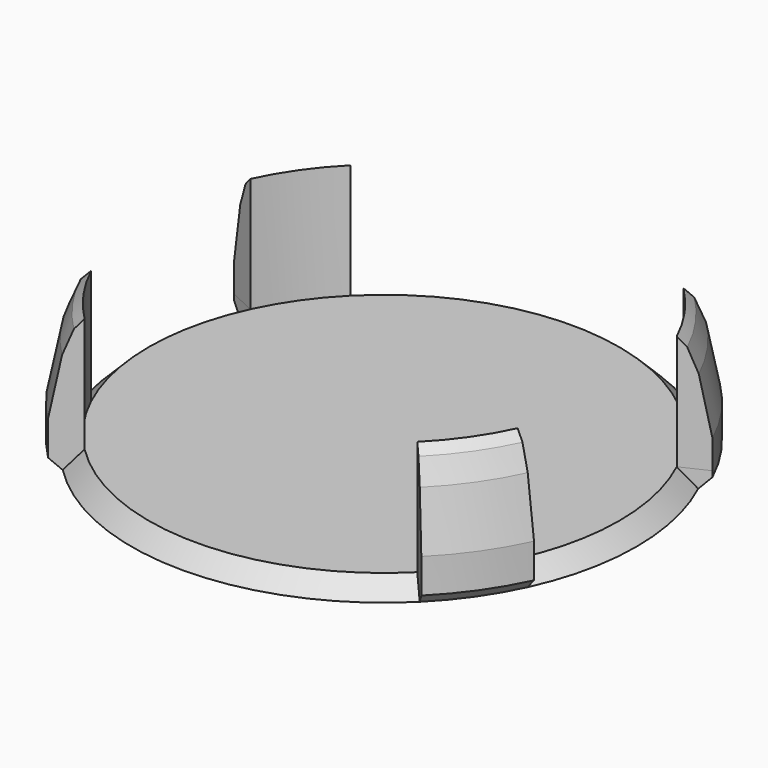
from build123d import *
from build123d import SkipClean  # not in build123d's __all__

# Parameters (mm, degrees)
F1_DEPTH    = 20
F2_SIZE     = 4.99999
F2_2_SIZE   = 4.99999
F2_3_SIZE   = 4.99999
F2_4_SIZE   = 4.99999
F3_DEPTH    = 3
F4_SIZE     = 5
F5_R        = 41
F5_R_2      = 39.2
F6_DEPTH    = 1.5
F7_SIZE     = 5
F8_T2_ANGLE = 50
F8_T4_ANGLE = 90
F8_T6_ANGLE = 50
F8_T8_ANGLE = 90
F9_SIZE     = 2


# Not quite as in the source:
# - a fillet or chamfer that OpenCascade refuses, or shapes differently, is made with other operations: its cross-section is extruded or revolved along the edge and cut away or added
# - a fillet or chamfer is up to 0.001 mm smaller than in the source, because OpenCascade refuses the exact size


with BuildPart() as f1:
    # F0 (on Top) → F1 (new body)
    with BuildSketch(Plane.XY):
        with BuildLine():
            ThreePointArc((-37.1586192685, 17.3273487314), (-33.5852338158, 23.5166338904), (-28.9913780286, 28.9913780286))
            Line((-28.9913780286, 28.9913780286), (-32.5269119346, 32.5269119346))
            ThreePointArc((-32.5269119346, 32.5269119346), (-37.6809940373, 26.3845160721), (-41.6901582037, 19.4404400401))
            Line((-41.6901582037, 19.4404400401), (-37.1586192685, 17.3273487314))
        make_face()
    extrude(amount=F1_DEPTH)

    # F2 (size 5 in the source; OpenCascade refuses exactly that, so slightly less here)
    f2_edges = [f1.edges().sort_by_distance(p)[0] for p in [
        (-37.680994, 26.384516, 20),
    ]]
    chamfer(f2_edges, length=F2_SIZE)



with BuildPart() as f1b:
    # F0 (on Top) → F1, piece 2 (new body)
    with BuildSketch(Plane.XY):
        with BuildLine():
            ThreePointArc((28.9913780286, 28.9913780286), (33.5852338158, 23.5166338904), (37.1586192685, 17.3273487314))
            Line((37.1586192685, 17.3273487314), (41.6901582037, 19.4404400401))
            ThreePointArc((41.6901582037, 19.4404400401), (37.6809940373, 26.3845160721), (32.5269119346, 32.5269119346))
            Line((32.5269119346, 32.5269119346), (28.9913780286, 28.9913780286))
        make_face()
    extrude(amount=F1_DEPTH)

    # F2#2 (size 5 in the source; OpenCascade refuses exactly that, so slightly less here)
    f2_2_edges = [f1b.edges().sort_by_distance(p)[0] for p in [
        (37.680994, 26.384516, 20),
    ]]
    chamfer(f2_2_edges, length=F2_2_SIZE)


with BuildPart() as f1c:
    # F0 (on Top) → F1, piece 3 (new body)
    with BuildSketch(Plane.XY):
        with BuildLine():
            Line((-32.5269119346, -32.5269119346), (-28.9913780286, -28.9913780286))
            ThreePointArc((-28.9913780286, -28.9913780286), (-33.5852338158, -23.5166338904), (-37.1586192685, -17.3273487314))
            Line((-37.1586192685, -17.3273487314), (-41.6901582037, -19.4404400401))
            ThreePointArc((-41.6901582037, -19.4404400401), (-37.6809940373, -26.3845160721), (-32.5269119346, -32.5269119346))
        make_face()
    extrude(amount=F1_DEPTH)

    # F2#3 (size 5 in the source; OpenCascade refuses exactly that, so slightly less here)
    f2_3_edges = [f1c.edges().sort_by_distance(p)[0] for p in [
        (-37.680994, -26.384516, 20),
    ]]
    chamfer(f2_3_edges, length=F2_3_SIZE)


with BuildPart() as f1d:
    # F0 (on Top) → F1, piece 4 (new body)
    with BuildSketch(Plane.XY):
        with BuildLine():
            Line((41.6901582037, -19.4404400401), (37.1586192685, -17.3273487314))
            ThreePointArc((37.1586192685, -17.3273487314), (33.5852338158, -23.5166338904), (28.9913780286, -28.9913780286))
            Line((28.9913780286, -28.9913780286), (32.5269119346, -32.5269119346))
            ThreePointArc((32.5269119346, -32.5269119346), (37.6809940373, -26.3845160721), (41.6901582037, -19.4404400401))
        make_face()
    extrude(amount=F1_DEPTH)

    # F2#4 (size 5 in the source; OpenCascade refuses exactly that, so slightly less here)
    f2_4_edges = [f1d.edges().sort_by_distance(p)[0] for p in [
        (37.680994, -26.384516, 20),
    ]]
    chamfer(f2_4_edges, length=F2_4_SIZE)


with BuildPart() as f1_1:
    add(f1.part, clean=False)

    with SkipClean():  # cleaning this boolean's faces spoils the solid; the shape is the same uncleaned
        add(f1b.part)  # F3 merges F1b

    with SkipClean():  # cleaning this boolean's faces spoils the solid; the shape is the same uncleaned
        add(f1c.part)  # F3 merges F1c

    with SkipClean():  # cleaning this boolean's faces spoils the solid; the shape is the same uncleaned
        add(f1d.part)  # F3 merges F1d
    # F0 (on Top) → F3 (join)
    with BuildSketch(Plane.XY):
        with BuildLine():
            ThreePointArc((-37.1586192685, 17.3273487314), (-33.5852338158, 23.5166338904), (-28.9913780286, 28.9913780286))
            Line((-28.9913780286, 28.9913780286), (-32.5269119346, 32.5269119346))
            ThreePointArc((-32.5269119346, 32.5269119346), (-37.6809940373, 26.3845160721), (-41.6901582037, 19.4404400401))
            Line((-41.6901582037, 19.4404400401), (-37.1586192685, 17.3273487314))
        make_face()
        with BuildLine():
            Line((32.5269119346, -32.5269119346), (28.9913780286, -28.9913780286))
            ThreePointArc((28.9913780286, -28.9913780286), (0, -41), (-28.9913780286, -28.9913780286))
            Line((-28.9913780286, -28.9913780286), (-32.5269119346, -32.5269119346))
            ThreePointArc((-32.5269119346, -32.5269119346), (0, -46), (32.5269119346, -32.5269119346))
        make_face()
        with BuildLine():
            ThreePointArc((28.9913780286, 28.9913780286), (33.5852338158, 23.5166338904), (37.1586192685, 17.3273487314))
            Line((37.1586192685, 17.3273487314), (41.6901582037, 19.4404400401))
            ThreePointArc((41.6901582037, 19.4404400401), (37.6809940373, 26.3845160721), (32.5269119346, 32.5269119346))
            Line((32.5269119346, 32.5269119346), (28.9913780286, 28.9913780286))
        make_face()
        with BuildLine():
            ThreePointArc((-28.9913780286, 28.9913780286), (0, 41), (28.9913780286, 28.9913780286))
            Line((28.9913780286, 28.9913780286), (32.5269119346, 32.5269119346))
            ThreePointArc((32.5269119346, 32.5269119346), (0, 46), (-32.5269119346, 32.5269119346))
            Line((-32.5269119346, 32.5269119346), (-28.9913780286, 28.9913780286))
        make_face()
        with BuildLine():
            ThreePointArc((37.1586192685, -17.3273487314), (40.0281362919, -8.8740241715), (41, 0))
            ThreePointArc((41, 0), (40.0281362919, 8.8740241715), (37.1586192685, 17.3273487314))
            ThreePointArc((37.1586192685, 17.3273487314), (33.5852338158, 23.5166338904), (28.9913780286, 28.9913780286))
            ThreePointArc((28.9913780286, 28.9913780286), (0, 41), (-28.9913780286, 28.9913780286))
            ThreePointArc((-28.9913780286, 28.9913780286), (-33.5852338158, 23.5166338904), (-37.1586192685, 17.3273487314))
            ThreePointArc((-37.1586192685, 17.3273487314), (-41, 0), (-37.1586192685, -17.3273487314))
            ThreePointArc((-37.1586192685, -17.3273487314), (-33.5852338158, -23.5166338904), (-28.9913780286, -28.9913780286))
            ThreePointArc((-28.9913780286, -28.9913780286), (0, -41), (28.9913780286, -28.9913780286))
            ThreePointArc((28.9913780286, -28.9913780286), (33.5852338158, -23.5166338904), (37.1586192685, -17.3273487314))
        make_face()
        with BuildLine():
            Line((-32.5269119346, -32.5269119346), (-28.9913780286, -28.9913780286))
            ThreePointArc((-28.9913780286, -28.9913780286), (-33.5852338158, -23.5166338904), (-37.1586192685, -17.3273487314))
            Line((-37.1586192685, -17.3273487314), (-41.6901582037, -19.4404400401))
            ThreePointArc((-41.6901582037, -19.4404400401), (-37.6809940373, -26.3845160721), (-32.5269119346, -32.5269119346))
        make_face()
        with BuildLine():
            Line((41.6901582037, -19.4404400401), (37.1586192685, -17.3273487314))
            ThreePointArc((37.1586192685, -17.3273487314), (33.5852338158, -23.5166338904), (28.9913780286, -28.9913780286))
            Line((28.9913780286, -28.9913780286), (32.5269119346, -32.5269119346))
            ThreePointArc((32.5269119346, -32.5269119346), (37.6809940373, -26.3845160721), (41.6901582037, -19.4404400401))
        make_face()
        with BuildLine():
            ThreePointArc((37.1586192685, 17.3273487314), (40.0281362919, 8.8740241715), (41, 0))
            ThreePointArc((41, 0), (40.0281362919, -8.8740241715), (37.1586192685, -17.3273487314))
            Line((37.1586192685, -17.3273487314), (41.6901582037, -19.4404400401))
            ThreePointArc((41.6901582037, -19.4404400401), (44.9096163275, -9.9562222412), (46, 0))
            ThreePointArc((46, 0), (44.9096163275, 9.9562222412), (41.6901582037, 19.4404400401))
            Line((41.6901582037, 19.4404400401), (37.1586192685, 17.3273487314))
        make_face()
        with BuildLine():
            ThreePointArc((-37.1586192685, -17.3273487314), (-41, 0), (-37.1586192685, 17.3273487314))
            Line((-37.1586192685, 17.3273487314), (-41.6901582037, 19.4404400401))
            ThreePointArc((-41.6901582037, 19.4404400401), (-46, 0), (-41.6901582037, -19.4404400401))
            Line((-41.6901582037, -19.4404400401), (-37.1586192685, -17.3273487314))
        make_face()
    with SkipClean():  # cleaning this boolean's faces spoils the solid; the shape is the same uncleaned
        extrude(amount=-F3_DEPTH)

    # F4
    f4_edges = [f1_1.edges().sort_by_distance(p)[0] for p in [
        (-37.680994, -26.384516, 15.00001),
        (-37.680994, 26.384516, 15.00001),
        (37.680994, -26.384516, 15.00001),
        (37.680994, 26.384516, 15.00001),
    ]]
    chamfer(f4_edges, length=F4_SIZE)

    # F5 (on face) → F6 (cut)
    with BuildSketch(Plane(origin=(0, 0, -3), x_dir=(1, 0, 0), z_dir=(0, 0, -1))):
        Circle(F5_R)
        Circle(F5_R_2, mode=Mode.SUBTRACT)
    with SkipClean():  # cleaning this boolean's faces spoils the solid; the shape is the same uncleaned
        extrude(amount=-F6_DEPTH, mode=Mode.SUBTRACT)

    # F7
    f7_edges = [f1_1.edges().sort_by_distance(p)[0] for p in [
        (-37.680994, -26.384516, 10.00001),
        (37.680994, -26.384516, 10.00001),
        (37.680994, 26.384516, 10.00001),
        (-37.680994, 26.384516, 10.00001),
    ]]
    chamfer(f7_edges, length=F7_SIZE)

    # F8: chamfer of 5 on 4 edges, made by hand

    # F8_s1 → F8_t2 (revolve, cut)
    with BuildSketch(Plane(origin=(0, 0, 0), x_dir=(0, 0, 1), z_dir=(0.4226182617, 0.906307787, 0))):
        Polygon((0, -41), (-5, -46), (0, -46), align=None)
    revolve(axis=Axis((0, 0, 0), (0, 0, 1)), revolution_arc=F8_T2_ANGLE, mode=Mode.SUBTRACT)

    # F8_s3 → F8_t4 (revolve, cut)
    with BuildSketch(Plane(origin=(0, 0, 0), x_dir=(0, 0, 1), z_dir=(0.7071067812, -0.7071067812, 0))):
        Polygon((0, -41), (-5, -46), (0, -46), align=None)
    revolve(axis=Axis((0, 0, 0), (0, 0, 1)), revolution_arc=F8_T4_ANGLE, mode=Mode.SUBTRACT)

    # F8_s5 → F8_t6 (revolve, cut)
    with BuildSketch(Plane(origin=(0, 0, 0), x_dir=(0, 0, 1), z_dir=(-0.4226182617, -0.906307787, 0))):
        Polygon((0, -41), (-5, -46), (0, -46), align=None)
    revolve(axis=Axis((0, 0, 0), (0, 0, 1)), revolution_arc=F8_T6_ANGLE, mode=Mode.SUBTRACT)

    # F8_s7 → F8_t8 (revolve, cut)
    with BuildSketch(Plane(origin=(0, 0, 0), x_dir=(0, 0, 1), z_dir=(-0.7071067812, 0.7071067812, 0))):
        Polygon((0, -41), (-5, -46), (0, -46), align=None)
    revolve(axis=Axis((0, 0, 0), (0, 0, 1)), revolution_arc=F8_T8_ANGLE, mode=Mode.SUBTRACT)

    # F9
    f9_edges = [f1_1.edges().sort_by_distance(p)[0] for p in [
        (-37.680994, -26.384516, -3),
        (37.680994, -26.384516, -3),
        (37.680994, 26.384516, -3),
        (-37.680994, 26.384516, -3),
    ]]
    chamfer(f9_edges, length=F9_SIZE)


solid = f1_1.part
